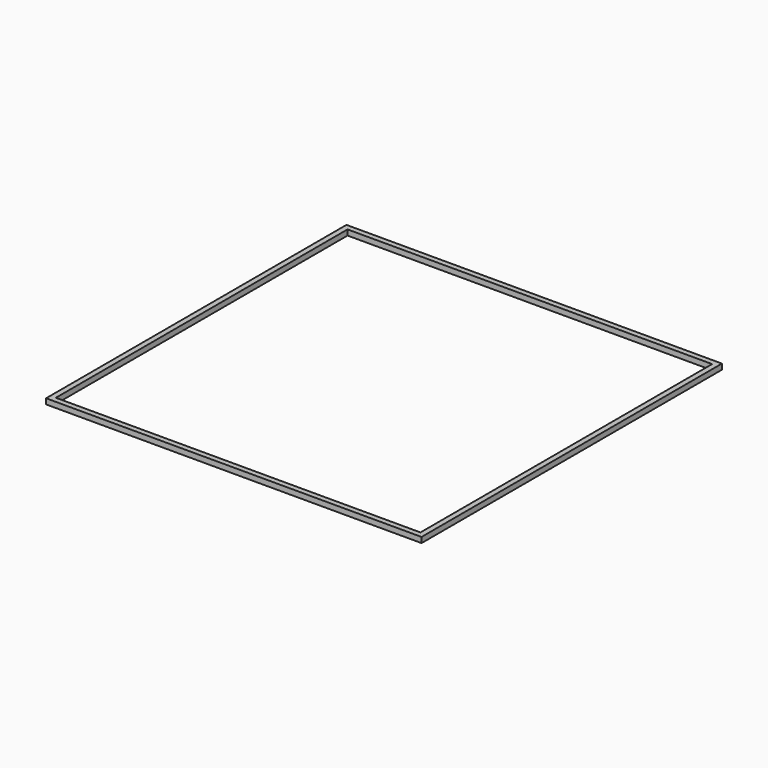
from build123d import *

# Parameters (mm, degrees)
F0_W     = 438.1
F0_H     = 438.1
F0_W_2   = 425.4
F0_H_2   = 425.4
F1_DEPTH = 6.35


# Not quite as in the source:
# - a length typed as a fraction of an inch, garbled in the dataset ("3 / 203.2 mm" for 3/8 in), is restored


with BuildPart() as f1:
    # F0 (on Top) → F1 (new body)
    with BuildSketch(Plane.XY):
        Rectangle(F0_W, F0_H)
        Rectangle(F0_W_2, F0_H_2, mode=Mode.SUBTRACT)
    extrude(amount=F1_DEPTH)


solid = f1.part
